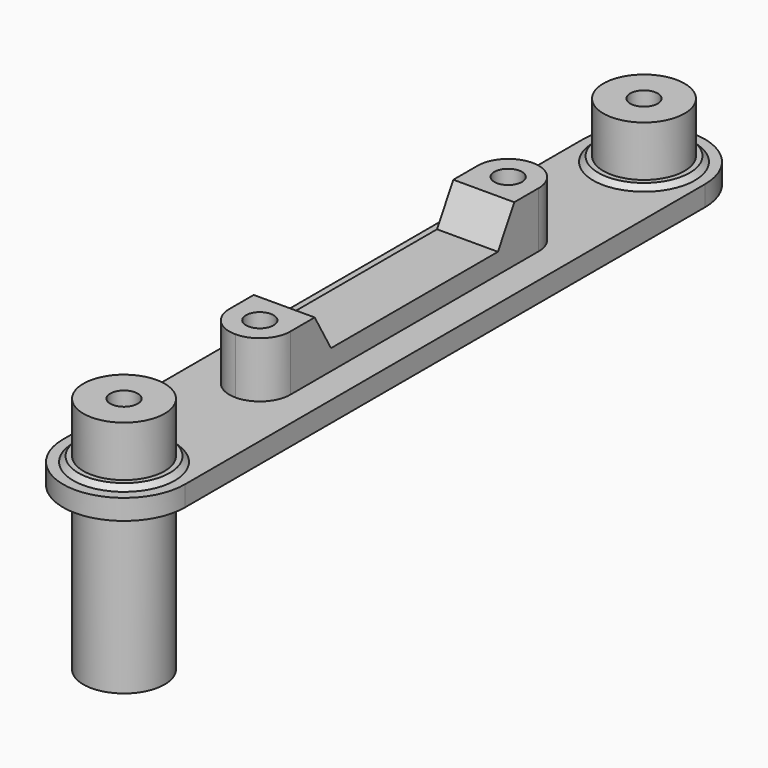
from build123d import *

# Parameters (mm, degrees)
F1_DEPTH       = 3.175
F2_W           = 9.525
F2_H           = 58.0526056528
F2_R           = 6.35
F3_DEPTH       = 8.6995
F5_DEPTH       = 9.525
F6_R           = 4.76249
F7_R           = 6.35
F8_DEPTH       = 25.4
F9_R           = 2.15265
F10_DEPTH      = 37.2745
F11_R          = 7.14375
F11_R_2        = 2.15265
F12_DEPTH      = 0.79375
F12_DEPTH_BACK = 3.96875
F13_R          = 7.14375
F13_R_2        = 2.15265
F14_DEPTH      = 0.79375
F15_SIZE       = 0.79374


# Not quite as in the source:
# - a fillet or chamfer is up to 0.001 mm smaller than in the source, because OpenCascade refuses the exact size


with BuildPart() as f1:
    # F0 (on Top) → F1 (new body)
    with BuildSketch(Plane.XY):
        with BuildLine():
            Line((0, 101.6), (0, 0))
            ThreePointArc((0, 0), (9.525, -9.525), (19.05, 0))
            Line((19.05, 0), (19.05, 101.6))
            ThreePointArc((19.05, 101.6), (9.525, 111.125), (0, 101.6))
        make_face()
    extrude(amount=F1_DEPTH)

    # F2 (on face) → F3 (join)
    with BuildSketch(Plane.XY.offset(3.175)):
        with Locations((9.525, 50.8)):
            Rectangle(F2_W, F2_H)
        with Locations((9.525, 0)):
            Circle(F2_R)
        with Locations((9.525, 101.6)):
            Circle(F2_R)
    extrude(amount=F3_DEPTH)

    # F4 (on face) → F5 (cut, through all)
    with BuildSketch(Plane(origin=(4.7625, 0, 0), x_dir=(0, -1, 0), z_dir=(-1, 0, 0))):
        Polygon((-34.4882687357, 6.35), (-31.2986971736, 11.8745), (-70.3013028264, 11.8745), (-67.1117312643, 6.35), align=None)
    extrude(amount=-F5_DEPTH, mode=Mode.SUBTRACT)

    # F6 (radius 4.7625 in the source; OpenCascade refuses exactly that, so slightly less here)
    f6_edges = [f1.edges().sort_by_distance(p)[0] for p in [
        (4.7625, 79.826303, 7.52475),
        (14.2875, 79.826303, 7.52475),
        (4.7625, 21.773697, 7.52475),
        (14.2875, 21.773697, 7.52475),
    ]]
    fillet(f6_edges, radius=F6_R)

    # F7 (on face) → F8 (join)
    with BuildSketch(Plane(origin=(0, 0, 0), x_dir=(1, 0, 0), z_dir=(0, 0, -1))):
        with Locations((9.525, 0)):
            Circle(F7_R)
    extrude(amount=F8_DEPTH)

    # F9 (on face) → F10 (cut, through all)
    with BuildSketch(Plane(origin=(0, 0, -25.4), x_dir=(1, 0, 0), z_dir=(0, 0, -1))):
        with Locations((9.525, 0)):
            Circle(F9_R)
        with Locations((9.525, -26.5361971736)):
            Circle(F9_R)
        with Locations((9.525, -75.0638028264)):
            Circle(F9_R)
        with Locations((9.525, -101.6)):
            Circle(F9_R)
    extrude(amount=-F10_DEPTH, mode=Mode.SUBTRACT)

    # F11 (on face) → F12 (join, two sides)
    with BuildSketch(Plane.XY.offset(3.175)) as f12_sk:
        with Locations((9.525, 0)):
            Circle(F11_R)
        with Locations((9.525, 0)):
            Circle(F11_R_2, mode=Mode.SUBTRACT)
    extrude(amount=F12_DEPTH)
    extrude(f12_sk.sketch, amount=-F12_DEPTH_BACK)

    # F13 (on face) → F14 (join, through all)
    with BuildSketch(Plane.XY.offset(3.175)):
        with Locations((9.525, 101.6)):
            Circle(F13_R)
        with Locations((9.525, 101.6)):
            Circle(F13_R_2, mode=Mode.SUBTRACT)
    extrude(amount=F14_DEPTH)

    # F15 (size 0.79375 in the source; OpenCascade refuses exactly that, so slightly less here)
    f15_edges = [f1.edges().sort_by_distance(p)[0] for p in [
        (2.38125, 101.6, 3.175),
        (2.38125, 0, 0),
        (2.38125, 0, 3.175),
    ]]
    chamfer(f15_edges, length=F15_SIZE)


solid = f1.part
